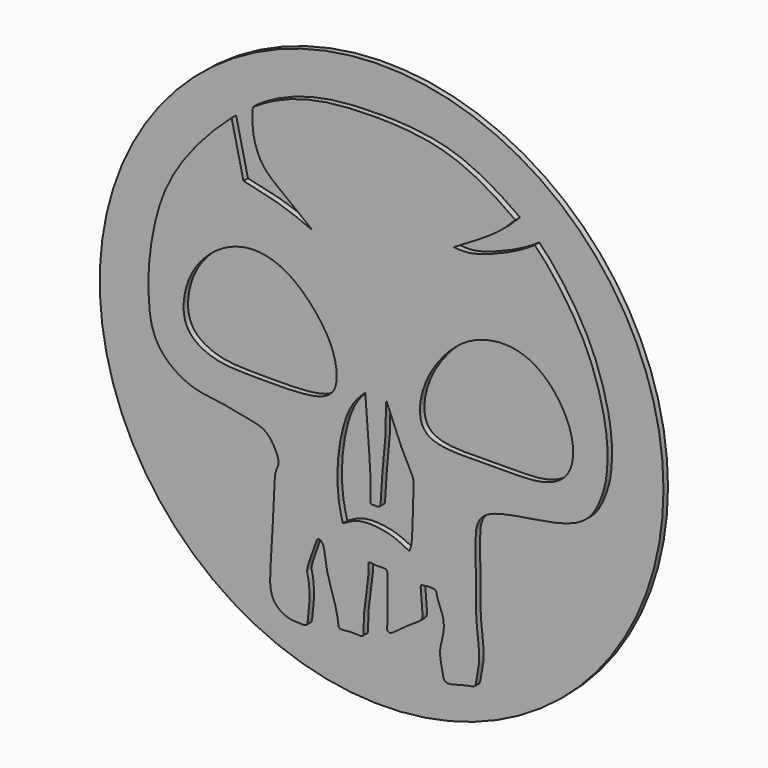
from build123d import *

# Parameters (mm, degrees)
F1_R     = 50
F2_DEPTH = 1
F3_DEPTH = 1


with BuildPart() as f2:
    # F1 (on Front) → F2 (new body)
    with BuildSketch(Plane.XZ):
        Circle(F1_R)
        with BuildLine():
            add(Edge.make_bspline(
                [(0, 42.2117872393), (-4.1518296289, 42.2328506159), (-11.7950982354, 41.7428127116), (-18.5583280025, 38.9956928302), (-21.8416117864, 36.8236386827), (-22.0455490568, 36.6854647788)],
                knots=[0, 0, 0, 0, 0.0225151774, 0.0438139107, 0.045228219, 0.045228219, 0.045228219, 0.045228219], degree=3))
            add(Edge.make_bspline(
                [(24.5358739047, 34.1949462892), (24.4433290355, 34.2621365821), (21.8294135785, 36.1505788176), (13.7200767318, 41.5241134747), (4.5021068795, 42.1889468096), (0, 42.2117872393)],
                knots=[0.9519222652, 0.9519222652, 0.9519222652, 0.9519222652, 0.9527753421, 0.9755852855, 1, 1, 1, 1], degree=3))
            add(Edge.make_bspline(
                [(27.9653905239, 31.395479857), (26.9777623389, 32.3428383748), (25.9556430174, 33.1641522159), (24.5358739047, 34.1949462892)],
                knots=[0.9388348597, 0.9388348597, 0.9388348597, 0.9388348597, 0.9519222652, 0.9519222652, 0.9519222652, 0.9519222652], degree=3))
            add(Edge.make_bspline(
                [(-25.8107159623, 33.7731806512), (-27.6085613015, 32.2136299029), (-32.3396448263, 27.4519948446), (-38.3374828793, 19.1153604845), (-40.6044889327, 7.5617746628), (-40.6895649134, 0.160899739), (-39.5035880323, -6.4994897033), (-33.3826669028, -10.9019134709), (-27.7631312299, -11.1810756086), (-22.678184549, -12.3446551948), (-19.2073445078, -12.8645914377), (-16.996587281, -17.3822862253), (-18.2265403297, -18.5991733267), (-18.3205187094, -24.5804643067), (-18.8558923982, -33.23684272), (-19.227253605, -39.2657426144), (-15.7491862761, -41.3032984762), (-13.6833573427, -41.1869410633), (-12.3461522337, -41.3189025592), (-12.259903056, -39.641815711), (-11.8422509257, -36.6374496799), (-12.1607198609, -33.5067173398), (-12.6847097019, -32.4134451461), (-11.0167872005, -28.3120606994), (-10.6319540152, -26.7097549158), (-9.2703902883, -27.4531554981), (-9.2454941531, -31.2745381629), (-7.1832623162, -36.42372276), (-6.8986091815, -39.104650667), (-6.7599340161, -39.930941303), (-5.1434315839, -39.5908424392), (-3.3777848263, -39.6631714956), (-2.3011178725, -39.7566957771), (-2.4275819303, -37.7459902706), (-2.3753767127, -35.3585257917), (-1.2109750063, -28.8526891406), (-1.7531941117, -27.5565836186), (-0.4279829764, -27.7785865503), (0.7443967174, -27.7854675929), (1.8262199292, -27.7259962358), (1.8186960843, -28.9119160062), (1.939885801, -36.3136478787), (1.7147514894, -37.153915214), (2.3153140554, -37.8653960955), (4.474137977, -35.7700630422), (7.9059440218, -33.949791946), (8.0597885263, -33.0338090974), (7.9964054591, -31.47586601), (7.5907060715, -28.3299618284), (8.0459994485, -28.1509086857), (10.0635743869, -27.9322750531), (10.5655419684, -28.4692820234), (10.6235516671, -29.4493784445), (12.046798778, -32.1975702095), (11.7372607804, -35.0029162994), (11.0287730808, -37.1627540966), (11.2943438203, -39.3279067847), (11.6822310138, -40.7688631927), (11.7641542089, -41.7336571667), (12.5927081487, -42.2437898456), (14.4897914582, -41.6547960008), (16.5386899479, -41.12852309), (17.497445307, -41.1386999382), (17.6748084447, -39.1404593024), (18.2501228287, -36.8914322934), (17.9208027823, -33.0181329788), (17.3852379788, -29.6683592104), (17.6574289505, -20.5026342529), (17.2814460979, -15.895420763), (19.3870938668, -12.641166496), (28.0889463204, -11.5115820335), (34.3484075669, -10.3351999916), (38.301085908, -7.8956922039), (40.1194286606, -3.4288857106), (40.8193777367, -0.4706351688), (41.1374570255, 6.3921409484), (37.8738587815, 18.2961121975), (32.0115398849, 26.9173704674), (29.2385585182, 30.1629197914), (28.0222448075, 31.3409437566), (27.9653905239, 31.395479857)],
                knots=[0.0541108044, 0.0541108044, 0.0541108044, 0.0541108044, 0.0671626411, 0.0900652708, 0.1122894062, 0.1301609437, 0.146680414, 0.1639138092, 0.1795682556, 0.194405388, 0.2065774387, 0.2200477559, 0.2278011522, 0.2432740409, 0.2633944941, 0.2788872676, 0.2909030042, 0.3003997174, 0.3070005619, 0.314507248, 0.3263972484, 0.3377885639, 0.3449893617, 0.3587443837, 0.3663284603, 0.3724509167, 0.3850088038, 0.4009612972, 0.4114994031, 0.4163389463, 0.4241766679, 0.4333217141, 0.439054527, 0.4471343161, 0.4581973396, 0.47507547, 0.4812862368, 0.4877545299, 0.4953651617, 0.5013243377, 0.5078482173, 0.5258276452, 0.5320393427, 0.5365745419, 0.5475076454, 0.5605446996, 0.5661163082, 0.5746275185, 0.5859814425, 0.5899877962, 0.5991364847, 0.6042707585, 0.6104528895, 0.6218419575, 0.6328992427, 0.6427529769, 0.6523553828, 0.6604165619, 0.666557621, 0.6722755539, 0.6815168022, 0.6912366323, 0.6968226628, 0.7053047419, 0.7156671247, 0.7281896012, 0.7406885031, 0.7605260422, 0.7746465306, 0.7862705734, 0.8054194498, 0.8223640938, 0.8360516094, 0.8499865894, 0.8613325091, 0.8780604221, 0.9013779912, 0.922684594, 0.9380814638, 0.9388348597, 0.9388348597, 0.9388348597, 0.9388348597], degree=3))
            add(Edge.make_bspline(
                [(-22.0455490568, 36.6854647788), (-23.3263802505, 35.8176614299), (-24.5871705589, 34.8345517868), (-25.8107159623, 33.7731806512)],
                knots=[0.045228219, 0.045228219, 0.045228219, 0.045228219, 0.0541108044, 0.0541108044, 0.0541108044, 0.0541108044], degree=3))
        make_face(mode=Mode.SUBTRACT)
        with BuildLine():
            add(Edge.make_bspline(
                [(24.5358739047, 34.1949462892), (24.4433290355, 34.2621365821), (21.8294135785, 36.1505788176), (13.7200767318, 41.5241134747), (4.5021068795, 42.1889468096), (0, 42.2117872393)],
                knots=[0.9519222652, 0.9519222652, 0.9519222652, 0.9519222652, 0.9527753421, 0.9755852855, 1, 1, 1, 1], degree=3))
            add(Edge.make_bspline(
                [(0, 42.2117872393), (-4.1518296289, 42.2328506159), (-11.7950982354, 41.7428127116), (-18.5583280025, 38.9956928302), (-21.8416117864, 36.8236386827), (-22.0455490568, 36.6854647788)],
                knots=[0, 0, 0, 0, 0.0225151774, 0.0438139107, 0.045228219, 0.045228219, 0.045228219, 0.045228219], degree=3))
            add(Edge.make_bspline(
                [(-11.4544853568, 20.8850093186), (-13.3831250096, 22.3815208443), (-16.8726422179, 25.0891840482), (-20.5810547116, 27.9211767393), (-22.2231186928, 32.4622663142), (-22.1061900395, 35.2963825837), (-22.0455490568, 36.6854647788)],
                knots=[0, 0, 0, 0, 0.294691905, 0.5330474492, 0.7706578355, 1, 1, 1, 1], degree=3))
            add(Edge.make_bspline(
                [(-23.7062107772, 24.6137939394), (-21.3903915949, 24.1204278596), (-16.9424193646, 23.1728242477), (-13.2327364884, 21.6263282704), (-11.4544853568, 20.8850093186)],
                knots=[0, 0, 0, 0, 0.5206460523, 1, 1, 1, 1], degree=3))
            add(Edge.make_bspline(
                [(-25.8107159623, 33.7731806512), (-25.1153904588, 30.7271716499), (-24.4015362806, 27.6598029406), (-23.7062107772, 24.6137939394)],
                knots=[0, 0, 0, 0, 9.3980480426, 9.3980480426, 9.3980480426, 9.3980480426], degree=3))
            add(Edge.make_bspline(
                [(-25.8107159623, 33.7731806512), (-27.6085613015, 32.2136299029), (-32.3396448263, 27.4519948446), (-38.3374828793, 19.1153604845), (-40.6044889327, 7.5617746628), (-40.6895649134, 0.160899739), (-39.5035880323, -6.4994897033), (-33.3826669028, -10.9019134709), (-27.7631312299, -11.1810756086), (-22.678184549, -12.3446551948), (-19.2073445078, -12.8645914377), (-16.996587281, -17.3822862253), (-18.2265403297, -18.5991733267), (-18.3205187094, -24.5804643067), (-18.8558923982, -33.23684272), (-19.227253605, -39.2657426144), (-15.7491862761, -41.3032984762), (-13.6833573427, -41.1869410633), (-12.3461522337, -41.3189025592), (-12.259903056, -39.641815711), (-11.8422509257, -36.6374496799), (-12.1607198609, -33.5067173398), (-12.6847097019, -32.4134451461), (-11.0167872005, -28.3120606994), (-10.6319540152, -26.7097549158), (-9.2703902883, -27.4531554981), (-9.2454941531, -31.2745381629), (-7.1832623162, -36.42372276), (-6.8986091815, -39.104650667), (-6.7599340161, -39.930941303), (-5.1434315839, -39.5908424392), (-3.3777848263, -39.6631714956), (-2.3011178725, -39.7566957771), (-2.4275819303, -37.7459902706), (-2.3753767127, -35.3585257917), (-1.2109750063, -28.8526891406), (-1.7531941117, -27.5565836186), (-0.4279829764, -27.7785865503), (0.7443967174, -27.7854675929), (1.8262199292, -27.7259962358), (1.8186960843, -28.9119160062), (1.939885801, -36.3136478787), (1.7147514894, -37.153915214), (2.3153140554, -37.8653960955), (4.474137977, -35.7700630422), (7.9059440218, -33.949791946), (8.0597885263, -33.0338090974), (7.9964054591, -31.47586601), (7.5907060715, -28.3299618284), (8.0459994485, -28.1509086857), (10.0635743869, -27.9322750531), (10.5655419684, -28.4692820234), (10.6235516671, -29.4493784445), (12.046798778, -32.1975702095), (11.7372607804, -35.0029162994), (11.0287730808, -37.1627540966), (11.2943438203, -39.3279067847), (11.6822310138, -40.7688631927), (11.7641542089, -41.7336571667), (12.5927081487, -42.2437898456), (14.4897914582, -41.6547960008), (16.5386899479, -41.12852309), (17.497445307, -41.1386999382), (17.6748084447, -39.1404593024), (18.2501228287, -36.8914322934), (17.9208027823, -33.0181329788), (17.3852379788, -29.6683592104), (17.6574289505, -20.5026342529), (17.2814460979, -15.895420763), (19.3870938668, -12.641166496), (28.0889463204, -11.5115820335), (34.3484075669, -10.3351999916), (38.301085908, -7.8956922039), (40.1194286606, -3.4288857106), (40.8193777367, -0.4706351688), (41.1374570255, 6.3921409484), (37.8738587815, 18.2961121975), (32.0115398849, 26.9173704674), (29.2385585182, 30.1629197914), (28.0222448075, 31.3409437566), (27.9653905239, 31.395479857)],
                knots=[0.0541108044, 0.0541108044, 0.0541108044, 0.0541108044, 0.0671626411, 0.0900652708, 0.1122894062, 0.1301609437, 0.146680414, 0.1639138092, 0.1795682556, 0.194405388, 0.2065774387, 0.2200477559, 0.2278011522, 0.2432740409, 0.2633944941, 0.2788872676, 0.2909030042, 0.3003997174, 0.3070005619, 0.314507248, 0.3263972484, 0.3377885639, 0.3449893617, 0.3587443837, 0.3663284603, 0.3724509167, 0.3850088038, 0.4009612972, 0.4114994031, 0.4163389463, 0.4241766679, 0.4333217141, 0.439054527, 0.4471343161, 0.4581973396, 0.47507547, 0.4812862368, 0.4877545299, 0.4953651617, 0.5013243377, 0.5078482173, 0.5258276452, 0.5320393427, 0.5365745419, 0.5475076454, 0.5605446996, 0.5661163082, 0.5746275185, 0.5859814425, 0.5899877962, 0.5991364847, 0.6042707585, 0.6104528895, 0.6218419575, 0.6328992427, 0.6427529769, 0.6523553828, 0.6604165619, 0.666557621, 0.6722755539, 0.6815168022, 0.6912366323, 0.6968226628, 0.7053047419, 0.7156671247, 0.7281896012, 0.7406885031, 0.7605260422, 0.7746465306, 0.7862705734, 0.8054194498, 0.8223640938, 0.8360516094, 0.8499865894, 0.8613325091, 0.8780604221, 0.9013779912, 0.922684594, 0.9380814638, 0.9388348597, 0.9388348597, 0.9388348597, 0.9388348597], degree=3))
            add(Edge.make_bspline(
                [(13.6259915307, 26.4096427709), (14.868920669, 26.2986663729), (17.2514108839, 26.1584062189), (24.774652777, 29.2598838581), (27.0484131927, 30.7945864143), (27.9653905239, 31.395479857)],
                knots=[0, 0, 0, 0, 0.2858529991, 0.7063590813, 1, 1, 1, 1], degree=3))
            add(Edge.make_bspline(
                [(24.5358739047, 34.1949462892), (23.4879896951, 33.0264970783), (20.5495068901, 30.4222182975), (16.2970825885, 28.0345928893), (13.6259915307, 26.4096427709)],
                knots=[0, 0, 0, 0, 0.442597588, 1, 1, 1, 1], degree=3))
        make_face()
        with BuildLine():
            add(Edge.make_bspline(
                [(-2.1085075568, -1.3914147858), (-3.0655404836, -2.3386562763), (-5.5176771557, -4.7964180048), (-7.3450347709, -13.6700454772), (-6.8720338251, -20.1809438225), (-6.3022172592, -22.2871682189), (-6.0797305778, -23.1139957905)],
                knots=[0, 0, 0, 0, 0.2268235626, 0.5470060722, 0.8206682651, 1, 1, 1, 1], degree=3))
            add(Edge.make_bspline(
                [(1.6345615732, -1.4169309288), (1.490965324, -2.8579625684), (1.6698736726, -6.4929197922), (0.9107367519, -12.0917960968), (0.6636329535, -17.6207516228), (0.5351646096, -18.5518819855), (-0.5243314009, -18.4901924912), (-1.3020890252, -18.5600471583), (-1.0587853603, -17.0466885783), (-1.1918373245, -12.325085245), (-1.738616593, -7.0220474396), (-1.9139538894, -3.1950838865), (-2.1085075568, -1.3914147858)],
                knots=[0, 0, 0, 0, 0.1261947039, 0.26822284, 0.4000888499, 0.4464504861, 0.5016773906, 0.5452860405, 0.6054317293, 0.7298231859, 0.865007954, 1, 1, 1, 1], degree=3))
            add(Edge.make_bspline(
                [(5.6894281879, -23.6325524747), (6.0294169274, -23.0262918846), (6.3029405429, -21.2201590976), (6.3502553341, -15.1137353852), (6.6592869733, -12.2924128873), (5.6112064851, -10.5424236095), (3.928762237, -7.2454551493), (2.4641075989, -3.3296749739), (1.6345615732, -1.4169309288)],
                knots=[0, 0, 0, 0, 0.135285802, 0.3516949921, 0.4971104265, 0.6137421047, 0.7799950182, 1, 1, 1, 1], degree=3))
            add(Edge.make_bspline(
                [(-6.0797305778, -23.1139957905), (-5.2821336221, -22.6623060144), (-3.6182047793, -21.7144926982), (-0.5535468195, -21.5575389799), (2.8281198488, -22.13058005), (4.8519182444, -23.1744974538), (5.6894281879, -23.6325524747)],
                knots=[0, 0, 0, 0, 0.2364754365, 0.4826011482, 0.746859744, 1, 1, 1, 1], degree=3))
        make_face(mode=Mode.SUBTRACT)
        with BuildLine():
            add(Edge.make_bspline(
                [(-22.5164033473, 14.4161963835), (-20.3056495064, 14.5739696965), (-15.4484858005, 13.3950084417), (-9.5326219645, 7.0982389572), (-7.1356121774, 2.062845141), (-6.9678023394, -3.1505079616), (-11.089146518, -5.5142723572), (-21.5012962295, -5.2798109014), (-28.3301322656, -5.4011257214), (-33.4486923273, -2.8583619411), (-34.7708764838, 1.3541160099), (-33.3589073398, 7.4905291071), (-28.777927567, 12.6107787217), (-24.6418312895, 14.2645124639), (-22.5164033473, 14.4161963835)],
                knots=[0, 0, 0, 0, 0.0881708155, 0.1857505695, 0.2659278088, 0.3368364609, 0.4040378762, 0.5125763687, 0.6028363001, 0.6783990179, 0.7453411296, 0.8279473944, 0.9152322111, 1, 1, 1, 1], degree=3))
        make_face(mode=Mode.SUBTRACT)
        with BuildLine():
            add(Edge.make_bspline(
                [(23.0282414705, 14.1640426591), (20.6607105304, 14.283315886), (15.4573377902, 13.0131761992), (10.31799426, 7.3226457935), (7.8487509767, 2.4597974628), (7.2390637852, -2.6959434398), (10.0779558768, -6.0752341115), (21.2791142164, -5.323258849), (28.6496767132, -5.8063992171), (34.0231438718, -3.4327860627), (35.2164049867, 1.6282631307), (33.614011723, 7.1077034989), (29.2591111394, 12.5282611205), (25.2107117158, 14.054092557), (23.0282414705, 14.1640426591)],
                knots=[0, 0, 0, 0, 0.0911618856, 0.1827766253, 0.2616710357, 0.3345437506, 0.3973678532, 0.5076618027, 0.6020481042, 0.6776726552, 0.7495279, 0.8289506007, 0.9159638848, 1, 1, 1, 1], degree=3))
        make_face(mode=Mode.SUBTRACT)
        with BuildLine():
            add(Edge.make_bspline(
                [(23.0282414705, 14.1640426591), (20.6607105304, 14.283315886), (15.4573377902, 13.0131761992), (10.31799426, 7.3226457935), (7.8487509767, 2.4597974628), (7.2390637852, -2.6959434398), (10.0779558768, -6.0752341115), (21.2791142164, -5.323258849), (28.6496767132, -5.8063992171), (34.0231438718, -3.4327860627), (35.2164049867, 1.6282631307), (33.614011723, 7.1077034989), (29.2591111394, 12.5282611205), (25.2107117158, 14.054092557), (23.0282414705, 14.1640426591)],
                knots=[0, 0, 0, 0, 0.0911618856, 0.1827766253, 0.2616710357, 0.3345437506, 0.3973678532, 0.5076618027, 0.6020481042, 0.6776726552, 0.7495279, 0.8289506007, 0.9159638848, 1, 1, 1, 1], degree=3))
        make_face()
        with BuildLine():
            add(Edge.make_bspline(
                [(-22.5164033473, 14.4161963835), (-20.3056495064, 14.5739696965), (-15.4484858005, 13.3950084417), (-9.5326219645, 7.0982389572), (-7.1356121774, 2.062845141), (-6.9678023394, -3.1505079616), (-11.089146518, -5.5142723572), (-21.5012962295, -5.2798109014), (-28.3301322656, -5.4011257214), (-33.4486923273, -2.8583619411), (-34.7708764838, 1.3541160099), (-33.3589073398, 7.4905291071), (-28.777927567, 12.6107787217), (-24.6418312895, 14.2645124639), (-22.5164033473, 14.4161963835)],
                knots=[0, 0, 0, 0, 0.0881708155, 0.1857505695, 0.2659278088, 0.3368364609, 0.4040378762, 0.5125763687, 0.6028363001, 0.6783990179, 0.7453411296, 0.8279473944, 0.9152322111, 1, 1, 1, 1], degree=3))
        make_face()
        with BuildLine():
            add(Edge.make_bspline(
                [(1.6345615732, -1.4169309288), (1.490965324, -2.8579625684), (1.6698736726, -6.4929197922), (0.9107367519, -12.0917960968), (0.6636329535, -17.6207516228), (0.5351646096, -18.5518819855), (-0.5243314009, -18.4901924912), (-1.3020890252, -18.5600471583), (-1.0587853603, -17.0466885783), (-1.1918373245, -12.325085245), (-1.738616593, -7.0220474396), (-1.9139538894, -3.1950838865), (-2.1085075568, -1.3914147858)],
                knots=[0, 0, 0, 0, 0.1261947039, 0.26822284, 0.4000888499, 0.4464504861, 0.5016773906, 0.5452860405, 0.6054317293, 0.7298231859, 0.865007954, 1, 1, 1, 1], degree=3))
            add(Edge.make_bspline(
                [(-2.1085075568, -1.3914147858), (-3.0655404836, -2.3386562763), (-5.5176771557, -4.7964180048), (-7.3450347709, -13.6700454772), (-6.8720338251, -20.1809438225), (-6.3022172592, -22.2871682189), (-6.0797305778, -23.1139957905)],
                knots=[0, 0, 0, 0, 0.2268235626, 0.5470060722, 0.8206682651, 1, 1, 1, 1], degree=3))
            add(Edge.make_bspline(
                [(-6.0797305778, -23.1139957905), (-5.2821336221, -22.6623060144), (-3.6182047793, -21.7144926982), (-0.5535468195, -21.5575389799), (2.8281198488, -22.13058005), (4.8519182444, -23.1744974538), (5.6894281879, -23.6325524747)],
                knots=[0, 0, 0, 0, 0.2364754365, 0.4826011482, 0.746859744, 1, 1, 1, 1], degree=3))
            add(Edge.make_bspline(
                [(5.6894281879, -23.6325524747), (6.0294169274, -23.0262918846), (6.3029405429, -21.2201590976), (6.3502553341, -15.1137353852), (6.6592869733, -12.2924128873), (5.6112064851, -10.5424236095), (3.928762237, -7.2454551493), (2.4641075989, -3.3296749739), (1.6345615732, -1.4169309288)],
                knots=[0, 0, 0, 0, 0.135285802, 0.3516949921, 0.4971104265, 0.6137421047, 0.7799950182, 1, 1, 1, 1], degree=3))
        make_face()
        with BuildLine():
            add(Edge.make_bspline(
                [(-11.4544853568, 20.8850093186), (-13.3831250096, 22.3815208443), (-16.8726422179, 25.0891840482), (-20.5810547116, 27.9211767393), (-22.2231186928, 32.4622663142), (-22.1061900395, 35.2963825837), (-22.0455490568, 36.6854647788)],
                knots=[0, 0, 0, 0, 0.294691905, 0.5330474492, 0.7706578355, 1, 1, 1, 1], degree=3))
            add(Edge.make_bspline(
                [(-22.0455490568, 36.6854647788), (-23.3263802505, 35.8176614299), (-24.5871705589, 34.8345517868), (-25.8107159623, 33.7731806512)],
                knots=[0.045228219, 0.045228219, 0.045228219, 0.045228219, 0.0541108044, 0.0541108044, 0.0541108044, 0.0541108044], degree=3))
            add(Edge.make_bspline(
                [(-25.8107159623, 33.7731806512), (-25.1153904588, 30.7271716499), (-24.4015362806, 27.6598029406), (-23.7062107772, 24.6137939394)],
                knots=[0, 0, 0, 0, 9.3980480426, 9.3980480426, 9.3980480426, 9.3980480426], degree=3))
            add(Edge.make_bspline(
                [(-23.7062107772, 24.6137939394), (-21.3903915949, 24.1204278596), (-16.9424193646, 23.1728242477), (-13.2327364884, 21.6263282704), (-11.4544853568, 20.8850093186)],
                knots=[0, 0, 0, 0, 0.5206460523, 1, 1, 1, 1], degree=3))
        make_face()
        with BuildLine():
            add(Edge.make_bspline(
                [(27.9653905239, 31.395479857), (26.9777623389, 32.3428383748), (25.9556430174, 33.1641522159), (24.5358739047, 34.1949462892)],
                knots=[0.9388348597, 0.9388348597, 0.9388348597, 0.9388348597, 0.9519222652, 0.9519222652, 0.9519222652, 0.9519222652], degree=3))
            add(Edge.make_bspline(
                [(24.5358739047, 34.1949462892), (23.4879896951, 33.0264970783), (20.5495068901, 30.4222182975), (16.2970825885, 28.0345928893), (13.6259915307, 26.4096427709)],
                knots=[0, 0, 0, 0, 0.442597588, 1, 1, 1, 1], degree=3))
            add(Edge.make_bspline(
                [(13.6259915307, 26.4096427709), (14.868920669, 26.2986663729), (17.2514108839, 26.1584062189), (24.774652777, 29.2598838581), (27.0484131927, 30.7945864143), (27.9653905239, 31.395479857)],
                knots=[0, 0, 0, 0, 0.2858529991, 0.7063590813, 1, 1, 1, 1], degree=3))
        make_face()
    extrude(amount=-F2_DEPTH)


with BuildPart() as f3:
    # F1 (on Front) → F3 (new body)
    with BuildSketch(Plane.XZ):
        with BuildLine():
            add(Edge.make_bspline(
                [(24.5358739047, 34.1949462892), (24.4433290355, 34.2621365821), (21.8294135785, 36.1505788176), (13.7200767318, 41.5241134747), (4.5021068795, 42.1889468096), (0, 42.2117872393)],
                knots=[0.9519222652, 0.9519222652, 0.9519222652, 0.9519222652, 0.9527753421, 0.9755852855, 1, 1, 1, 1], degree=3))
            add(Edge.make_bspline(
                [(0, 42.2117872393), (-4.1518296289, 42.2328506159), (-11.7950982354, 41.7428127116), (-18.5583280025, 38.9956928302), (-21.8416117864, 36.8236386827), (-22.0455490568, 36.6854647788)],
                knots=[0, 0, 0, 0, 0.0225151774, 0.0438139107, 0.045228219, 0.045228219, 0.045228219, 0.045228219], degree=3))
            add(Edge.make_bspline(
                [(-11.4544853568, 20.8850093186), (-13.3831250096, 22.3815208443), (-16.8726422179, 25.0891840482), (-20.5810547116, 27.9211767393), (-22.2231186928, 32.4622663142), (-22.1061900395, 35.2963825837), (-22.0455490568, 36.6854647788)],
                knots=[0, 0, 0, 0, 0.294691905, 0.5330474492, 0.7706578355, 1, 1, 1, 1], degree=3))
            add(Edge.make_bspline(
                [(-23.7062107772, 24.6137939394), (-21.3903915949, 24.1204278596), (-16.9424193646, 23.1728242477), (-13.2327364884, 21.6263282704), (-11.4544853568, 20.8850093186)],
                knots=[0, 0, 0, 0, 0.5206460523, 1, 1, 1, 1], degree=3))
            add(Edge.make_bspline(
                [(-25.8107159623, 33.7731806512), (-25.1153904588, 30.7271716499), (-24.4015362806, 27.6598029406), (-23.7062107772, 24.6137939394)],
                knots=[0, 0, 0, 0, 9.3980480426, 9.3980480426, 9.3980480426, 9.3980480426], degree=3))
            add(Edge.make_bspline(
                [(-25.8107159623, 33.7731806512), (-27.6085613015, 32.2136299029), (-32.3396448263, 27.4519948446), (-38.3374828793, 19.1153604845), (-40.6044889327, 7.5617746628), (-40.6895649134, 0.160899739), (-39.5035880323, -6.4994897033), (-33.3826669028, -10.9019134709), (-27.7631312299, -11.1810756086), (-22.678184549, -12.3446551948), (-19.2073445078, -12.8645914377), (-16.996587281, -17.3822862253), (-18.2265403297, -18.5991733267), (-18.3205187094, -24.5804643067), (-18.8558923982, -33.23684272), (-19.227253605, -39.2657426144), (-15.7491862761, -41.3032984762), (-13.6833573427, -41.1869410633), (-12.3461522337, -41.3189025592), (-12.259903056, -39.641815711), (-11.8422509257, -36.6374496799), (-12.1607198609, -33.5067173398), (-12.6847097019, -32.4134451461), (-11.0167872005, -28.3120606994), (-10.6319540152, -26.7097549158), (-9.2703902883, -27.4531554981), (-9.2454941531, -31.2745381629), (-7.1832623162, -36.42372276), (-6.8986091815, -39.104650667), (-6.7599340161, -39.930941303), (-5.1434315839, -39.5908424392), (-3.3777848263, -39.6631714956), (-2.3011178725, -39.7566957771), (-2.4275819303, -37.7459902706), (-2.3753767127, -35.3585257917), (-1.2109750063, -28.8526891406), (-1.7531941117, -27.5565836186), (-0.4279829764, -27.7785865503), (0.7443967174, -27.7854675929), (1.8262199292, -27.7259962358), (1.8186960843, -28.9119160062), (1.939885801, -36.3136478787), (1.7147514894, -37.153915214), (2.3153140554, -37.8653960955), (4.474137977, -35.7700630422), (7.9059440218, -33.949791946), (8.0597885263, -33.0338090974), (7.9964054591, -31.47586601), (7.5907060715, -28.3299618284), (8.0459994485, -28.1509086857), (10.0635743869, -27.9322750531), (10.5655419684, -28.4692820234), (10.6235516671, -29.4493784445), (12.046798778, -32.1975702095), (11.7372607804, -35.0029162994), (11.0287730808, -37.1627540966), (11.2943438203, -39.3279067847), (11.6822310138, -40.7688631927), (11.7641542089, -41.7336571667), (12.5927081487, -42.2437898456), (14.4897914582, -41.6547960008), (16.5386899479, -41.12852309), (17.497445307, -41.1386999382), (17.6748084447, -39.1404593024), (18.2501228287, -36.8914322934), (17.9208027823, -33.0181329788), (17.3852379788, -29.6683592104), (17.6574289505, -20.5026342529), (17.2814460979, -15.895420763), (19.3870938668, -12.641166496), (28.0889463204, -11.5115820335), (34.3484075669, -10.3351999916), (38.301085908, -7.8956922039), (40.1194286606, -3.4288857106), (40.8193777367, -0.4706351688), (41.1374570255, 6.3921409484), (37.8738587815, 18.2961121975), (32.0115398849, 26.9173704674), (29.2385585182, 30.1629197914), (28.0222448075, 31.3409437566), (27.9653905239, 31.395479857)],
                knots=[0.0541108044, 0.0541108044, 0.0541108044, 0.0541108044, 0.0671626411, 0.0900652708, 0.1122894062, 0.1301609437, 0.146680414, 0.1639138092, 0.1795682556, 0.194405388, 0.2065774387, 0.2200477559, 0.2278011522, 0.2432740409, 0.2633944941, 0.2788872676, 0.2909030042, 0.3003997174, 0.3070005619, 0.314507248, 0.3263972484, 0.3377885639, 0.3449893617, 0.3587443837, 0.3663284603, 0.3724509167, 0.3850088038, 0.4009612972, 0.4114994031, 0.4163389463, 0.4241766679, 0.4333217141, 0.439054527, 0.4471343161, 0.4581973396, 0.47507547, 0.4812862368, 0.4877545299, 0.4953651617, 0.5013243377, 0.5078482173, 0.5258276452, 0.5320393427, 0.5365745419, 0.5475076454, 0.5605446996, 0.5661163082, 0.5746275185, 0.5859814425, 0.5899877962, 0.5991364847, 0.6042707585, 0.6104528895, 0.6218419575, 0.6328992427, 0.6427529769, 0.6523553828, 0.6604165619, 0.666557621, 0.6722755539, 0.6815168022, 0.6912366323, 0.6968226628, 0.7053047419, 0.7156671247, 0.7281896012, 0.7406885031, 0.7605260422, 0.7746465306, 0.7862705734, 0.8054194498, 0.8223640938, 0.8360516094, 0.8499865894, 0.8613325091, 0.8780604221, 0.9013779912, 0.922684594, 0.9380814638, 0.9388348597, 0.9388348597, 0.9388348597, 0.9388348597], degree=3))
            add(Edge.make_bspline(
                [(13.6259915307, 26.4096427709), (14.868920669, 26.2986663729), (17.2514108839, 26.1584062189), (24.774652777, 29.2598838581), (27.0484131927, 30.7945864143), (27.9653905239, 31.395479857)],
                knots=[0, 0, 0, 0, 0.2858529991, 0.7063590813, 1, 1, 1, 1], degree=3))
            add(Edge.make_bspline(
                [(24.5358739047, 34.1949462892), (23.4879896951, 33.0264970783), (20.5495068901, 30.4222182975), (16.2970825885, 28.0345928893), (13.6259915307, 26.4096427709)],
                knots=[0, 0, 0, 0, 0.442597588, 1, 1, 1, 1], degree=3))
        make_face()
        with BuildLine():
            add(Edge.make_bspline(
                [(-2.1085075568, -1.3914147858), (-3.0655404836, -2.3386562763), (-5.5176771557, -4.7964180048), (-7.3450347709, -13.6700454772), (-6.8720338251, -20.1809438225), (-6.3022172592, -22.2871682189), (-6.0797305778, -23.1139957905)],
                knots=[0, 0, 0, 0, 0.2268235626, 0.5470060722, 0.8206682651, 1, 1, 1, 1], degree=3))
            add(Edge.make_bspline(
                [(1.6345615732, -1.4169309288), (1.490965324, -2.8579625684), (1.6698736726, -6.4929197922), (0.9107367519, -12.0917960968), (0.6636329535, -17.6207516228), (0.5351646096, -18.5518819855), (-0.5243314009, -18.4901924912), (-1.3020890252, -18.5600471583), (-1.0587853603, -17.0466885783), (-1.1918373245, -12.325085245), (-1.738616593, -7.0220474396), (-1.9139538894, -3.1950838865), (-2.1085075568, -1.3914147858)],
                knots=[0, 0, 0, 0, 0.1261947039, 0.26822284, 0.4000888499, 0.4464504861, 0.5016773906, 0.5452860405, 0.6054317293, 0.7298231859, 0.865007954, 1, 1, 1, 1], degree=3))
            add(Edge.make_bspline(
                [(5.6894281879, -23.6325524747), (6.0294169274, -23.0262918846), (6.3029405429, -21.2201590976), (6.3502553341, -15.1137353852), (6.6592869733, -12.2924128873), (5.6112064851, -10.5424236095), (3.928762237, -7.2454551493), (2.4641075989, -3.3296749739), (1.6345615732, -1.4169309288)],
                knots=[0, 0, 0, 0, 0.135285802, 0.3516949921, 0.4971104265, 0.6137421047, 0.7799950182, 1, 1, 1, 1], degree=3))
            add(Edge.make_bspline(
                [(-6.0797305778, -23.1139957905), (-5.2821336221, -22.6623060144), (-3.6182047793, -21.7144926982), (-0.5535468195, -21.5575389799), (2.8281198488, -22.13058005), (4.8519182444, -23.1744974538), (5.6894281879, -23.6325524747)],
                knots=[0, 0, 0, 0, 0.2364754365, 0.4826011482, 0.746859744, 1, 1, 1, 1], degree=3))
        make_face(mode=Mode.SUBTRACT)
        with BuildLine():
            add(Edge.make_bspline(
                [(-22.5164033473, 14.4161963835), (-20.3056495064, 14.5739696965), (-15.4484858005, 13.3950084417), (-9.5326219645, 7.0982389572), (-7.1356121774, 2.062845141), (-6.9678023394, -3.1505079616), (-11.089146518, -5.5142723572), (-21.5012962295, -5.2798109014), (-28.3301322656, -5.4011257214), (-33.4486923273, -2.8583619411), (-34.7708764838, 1.3541160099), (-33.3589073398, 7.4905291071), (-28.777927567, 12.6107787217), (-24.6418312895, 14.2645124639), (-22.5164033473, 14.4161963835)],
                knots=[0, 0, 0, 0, 0.0881708155, 0.1857505695, 0.2659278088, 0.3368364609, 0.4040378762, 0.5125763687, 0.6028363001, 0.6783990179, 0.7453411296, 0.8279473944, 0.9152322111, 1, 1, 1, 1], degree=3))
        make_face(mode=Mode.SUBTRACT)
        with BuildLine():
            add(Edge.make_bspline(
                [(23.0282414705, 14.1640426591), (20.6607105304, 14.283315886), (15.4573377902, 13.0131761992), (10.31799426, 7.3226457935), (7.8487509767, 2.4597974628), (7.2390637852, -2.6959434398), (10.0779558768, -6.0752341115), (21.2791142164, -5.323258849), (28.6496767132, -5.8063992171), (34.0231438718, -3.4327860627), (35.2164049867, 1.6282631307), (33.614011723, 7.1077034989), (29.2591111394, 12.5282611205), (25.2107117158, 14.054092557), (23.0282414705, 14.1640426591)],
                knots=[0, 0, 0, 0, 0.0911618856, 0.1827766253, 0.2616710357, 0.3345437506, 0.3973678532, 0.5076618027, 0.6020481042, 0.6776726552, 0.7495279, 0.8289506007, 0.9159638848, 1, 1, 1, 1], degree=3))
        make_face(mode=Mode.SUBTRACT)
    extrude(amount=F3_DEPTH)


with BuildPart() as f2_1:
    # F4: moved
    add(f2.part)


solid = Compound([f3.part, f2_1.part])
